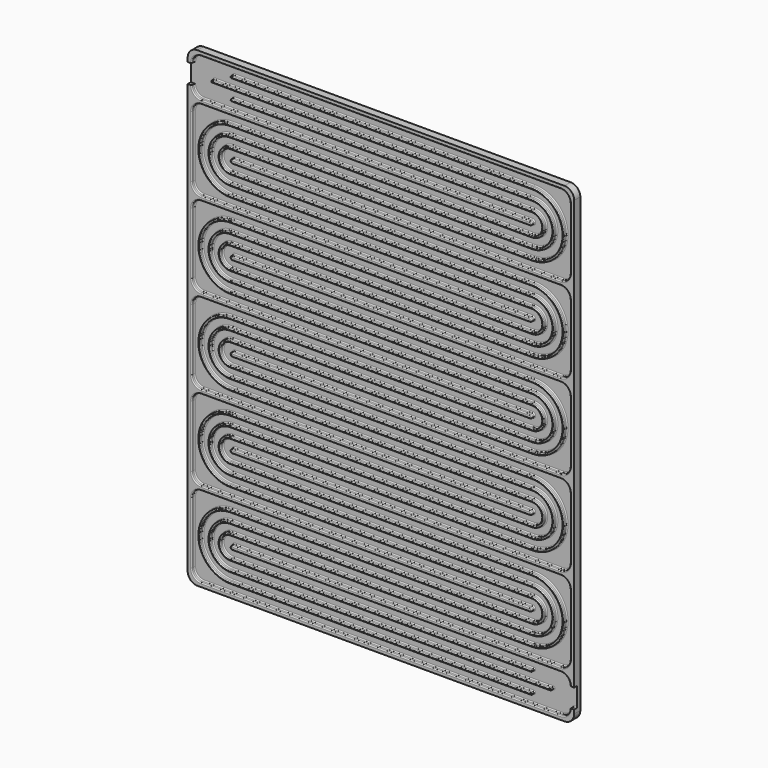
from build123d import *

# Parameters (mm, degrees)
F1_DEPTH = 4
F3_DEPTH = 2
F4_W     = 156
F4_H     = 1
F5_DEPTH = 2
F6_R     = 0.49999


# Not quite as in the source:
# - a fillet or chamfer is up to 0.001 mm smaller than in the source, because OpenCascade refuses the exact size


with BuildPart() as f1:
    # F0 (on Front) → F1 (new body)
    with BuildSketch(Plane.XZ):
        with BuildLine():
            ThreePointArc((0, 5), (1.4644660941, 1.4644660941), (5, 0))
            Line((5, 0), (195, 0))
            ThreePointArc((195, 0), (198.5355339059, 1.4644660941), (200, 5))
            Line((200, 5), (200, 239))
            ThreePointArc((200, 239), (198.5355339059, 242.5355339059), (195, 244))
            Line((195, 244), (5, 244))
            ThreePointArc((5, 244), (1.4644660941, 242.5355339059), (0, 239))
            Line((0, 239), (0, 5))
        make_face()
    extrude(amount=F1_DEPTH)

    # F2 (on face) → F3 (cut)
    with BuildSketch(Plane.XZ.offset(4)):
        with BuildLine():
            Line((193, 242), (7, 242))
            ThreePointArc((7, 242), (3.4644660941, 240.5355339059), (2, 237))
            Line((2, 237), (0, 237))
            Line((0, 237), (0, 227))
            Line((0, 227), (2, 227))
            ThreePointArc((2, 227), (3.4644660941, 223.4644660941), (7, 222))
            Line((7, 222), (177, 222))
            ThreePointArc((177, 222), (177.7071067812, 221.7071067812), (178, 221))
            ThreePointArc((178, 221), (177.7071067812, 220.2928932188), (177, 220))
            Line((177, 220), (7, 220))
            ThreePointArc((7, 220), (3.4644660941, 218.5355339059), (2, 215))
            Line((2, 215), (2, 183))
            ThreePointArc((2, 183), (3.4644660941, 179.4644660941), (7, 178))
            Line((7, 178), (177, 178))
            ThreePointArc((177, 178), (177.7071067812, 177.7071067812), (178, 177))
            ThreePointArc((178, 177), (177.7071067812, 176.2928932188), (177, 176))
            Line((177, 176), (7, 176))
            ThreePointArc((7, 176), (3.4644660941, 174.5355339059), (2, 171))
            Line((2, 171), (2, 139))
            ThreePointArc((2, 139), (3.4644660941, 135.4644660941), (7, 134))
            Line((7, 134), (177, 134))
            ThreePointArc((177, 134), (177.7071067812, 133.7071067812), (178, 133))
            ThreePointArc((178, 133), (177.7071067812, 132.2928932188), (177, 132))
            Line((177, 132), (7, 132))
            ThreePointArc((7, 132), (3.4644660941, 130.5355339059), (2, 127))
            Line((2, 127), (2, 95))
            ThreePointArc((2, 95), (3.4644660941, 91.4644660941), (7, 90))
            Line((7, 90), (177, 90))
            ThreePointArc((177, 90), (177.7071067812, 89.7071067812), (178, 89))
            ThreePointArc((178, 89), (177.7071067812, 88.2928932188), (177, 88))
            Line((177, 88), (7, 88))
            ThreePointArc((7, 88), (3.4644660941, 86.5355339059), (2, 83))
            Line((2, 83), (2, 51))
            ThreePointArc((2, 51), (3.4644660941, 47.4644660941), (7, 46))
            Line((7, 46), (177, 46))
            ThreePointArc((177, 46), (177.7071067812, 45.7071067812), (178, 45))
            ThreePointArc((178, 45), (177.7071067812, 44.2928932188), (177, 44))
            Line((177, 44), (6.8, 44))
            ThreePointArc((6.8, 44), (3.4058874503, 42.5941125497), (2, 39.2))
            Line((2, 39.2), (2, 7))
            ThreePointArc((2, 7), (3.4644660941, 3.4644660941), (7, 2))
            Line((7, 2), (193, 2))
            ThreePointArc((193, 2), (196.5355339059, 3.4644660941), (198, 7))
            Line((198, 7), (200, 7))
            Line((200, 7), (200, 17))
            Line((200, 17), (198, 17))
            ThreePointArc((198, 17), (196.5355339059, 20.5355339059), (193, 22))
            Line((193, 22), (23, 22))
            ThreePointArc((23, 22), (22.2928932188, 22.2928932188), (22, 23))
            ThreePointArc((22, 23), (22.2928932188, 23.7071067812), (23, 24))
            Line((23, 24), (193, 24))
            ThreePointArc((193, 24), (196.5355339059, 25.4644660941), (198, 29))
            Line((198, 29), (198, 61))
            ThreePointArc((198, 61), (196.5355339059, 64.5355339059), (193, 66))
            Line((193, 66), (23, 66))
            ThreePointArc((23, 66), (22.2928932188, 66.2928932188), (22, 67))
            ThreePointArc((22, 67), (22.2928932188, 67.7071067812), (23, 68))
            Line((23, 68), (193, 68))
            ThreePointArc((193, 68), (196.5355339059, 69.4644660941), (198, 73))
            Line((198, 73), (198, 105))
            ThreePointArc((198, 105), (196.5355339059, 108.5355339059), (193, 110))
            Line((193, 110), (23, 110))
            ThreePointArc((23, 110), (22.2928932188, 110.2928932188), (22, 111))
            ThreePointArc((22, 111), (22.2928932188, 111.7071067812), (23, 112))
            Line((23, 112), (193, 112))
            ThreePointArc((193, 112), (196.5355339059, 113.4644660941), (198, 117))
            Line((198, 117), (198, 149))
            ThreePointArc((198, 149), (196.5355339059, 152.5355339059), (193, 154))
            Line((193, 154), (23, 154))
            ThreePointArc((23, 154), (22.2928932188, 154.2928932188), (22, 155))
            ThreePointArc((22, 155), (22.2928932188, 155.7071067812), (23, 156))
            Line((23, 156), (193, 156))
            ThreePointArc((193, 156), (196.5355339059, 157.4644660941), (198, 161))
            Line((198, 161), (198, 193))
            ThreePointArc((198, 193), (196.5355339059, 196.5355339059), (193, 198))
            Line((193, 198), (23, 198))
            ThreePointArc((23, 198), (22.2928932188, 198.2928932188), (22, 199))
            ThreePointArc((22, 199), (22.2928932188, 199.7071067812), (23, 200))
            Line((23, 200), (193, 200))
            ThreePointArc((193, 200), (196.5355339059, 201.4644660941), (198, 205))
            Line((198, 205), (198, 237))
            ThreePointArc((198, 237), (196.5355339059, 240.5355339059), (193, 242))
        make_face()
    extrude(amount=-F3_DEPTH, mode=Mode.SUBTRACT)

    # F4 (on face) → F5 (join)
    with BuildSketch(Plane.XZ.offset(2)):
        with Locations((100, 6.75)):
            Rectangle(F4_W, F4_H)
        with BuildLine():
            Line((22, 6.25), (22, 7.25))
            ThreePointArc((22, 7.25), (6.25, 23), (22, 38.75))
            Line((22, 38.75), (178, 38.75))
            ThreePointArc((178, 38.75), (184.25, 45), (178, 51.25))
            Line((178, 51.25), (22, 51.25))
            Line((22, 51.25), (22, 50.25))
            Line((22, 50.25), (178, 50.25))
            ThreePointArc((178, 50.25), (183.25, 45), (178, 39.75))
            Line((178, 39.75), (22, 39.75))
            ThreePointArc((22, 39.75), (5.25, 23), (22, 6.25))
        make_face()
        with BuildLine():
            Line((22, 50.25), (22, 51.25))
            ThreePointArc((22, 51.25), (6.25, 67), (22, 82.75))
            Line((22, 82.75), (22, 83.75))
            ThreePointArc((22, 83.75), (5.25, 67), (22, 50.25))
        make_face()
        with Locations((100, 83.25)):
            Rectangle(F4_W, F4_H)
        with BuildLine():
            Line((178, 83.75), (178, 82.75))
            ThreePointArc((178, 82.75), (184.25, 89), (178, 95.25))
            Line((178, 95.25), (178, 94.25))
            ThreePointArc((178, 94.25), (183.25, 89), (178, 83.75))
        make_face()
        with Locations((100, 94.75)):
            Rectangle(F4_W, F4_H)
        with BuildLine():
            Line((22, 94.25), (22, 95.25))
            ThreePointArc((22, 95.25), (6.25, 111), (22, 126.75))
            Line((22, 126.75), (22, 127.75))
            ThreePointArc((22, 127.75), (5.25, 111), (22, 94.25))
        make_face()
        with Locations((100, 127.25)):
            Rectangle(F4_W, F4_H)
        with BuildLine():
            Line((178, 127.75), (178, 126.75))
            ThreePointArc((178, 126.75), (184.25, 133), (178, 139.25))
            Line((178, 139.25), (178, 138.25))
            ThreePointArc((178, 138.25), (183.25, 133), (178, 127.75))
        make_face()
        with Locations((100, 138.75)):
            Rectangle(F4_W, F4_H)
        with BuildLine():
            Line((22, 138.25), (22, 139.25))
            ThreePointArc((22, 139.25), (6.25, 155), (22, 170.75))
            Line((22, 170.75), (22, 171.75))
            ThreePointArc((22, 171.75), (5.25, 155), (22, 138.25))
        make_face()
        with Locations((100, 171.25)):
            Rectangle(F4_W, F4_H)
        with BuildLine():
            Line((178, 171.75), (178, 170.75))
            ThreePointArc((178, 170.75), (184.25, 177), (178, 183.25))
            Line((178, 183.25), (178, 182.25))
            ThreePointArc((178, 182.25), (183.25, 177), (178, 171.75))
        make_face()
        with Locations((100, 182.75)):
            Rectangle(F4_W, F4_H)
        with BuildLine():
            Line((22, 182.25), (22, 183.25))
            ThreePointArc((22, 183.25), (6.25, 199), (22, 214.75))
            Line((22, 214.75), (22, 215.75))
            ThreePointArc((22, 215.75), (5.25, 199), (22, 182.25))
        make_face()
        with Locations((100, 215.25)):
            Rectangle(F4_W, F4_H)
        with BuildLine():
            Line((178, 215.75), (178, 214.75))
            ThreePointArc((178, 214.75), (184.25, 221), (178, 227.25))
            Line((178, 227.25), (178, 226.25))
            ThreePointArc((178, 226.25), (183.25, 221), (178, 215.75))
        make_face()
        with Locations((100, 226.75)):
            Rectangle(F4_W, F4_H)
        Polygon((178, 12.5), (22, 12.5), (22, 11.5), (178, 11.5), (188, 11.5), (188, 12.5), align=None)
        with BuildLine():
            Line((22, 11.5), (22, 12.5))
            ThreePointArc((22, 12.5), (11.5, 23), (22, 33.5))
            Line((22, 33.5), (178, 33.5))
            ThreePointArc((178, 33.5), (189.5, 45), (178, 56.5))
            Line((178, 56.5), (22, 56.5))
            Line((22, 56.5), (22, 55.5))
            Line((22, 55.5), (178, 55.5))
            ThreePointArc((178, 55.5), (188.5, 45), (178, 34.5))
            Line((178, 34.5), (22, 34.5))
            ThreePointArc((22, 34.5), (10.5, 23), (22, 11.5))
        make_face()
        with BuildLine():
            Line((22, 55.5), (22, 56.5))
            ThreePointArc((22, 56.5), (11.5, 67), (22, 77.5))
            Line((22, 77.5), (22, 78.5))
            ThreePointArc((22, 78.5), (10.5, 67), (22, 55.5))
        make_face()
        with Locations((100, 78)):
            Rectangle(F4_W, F4_H)
        with BuildLine():
            Line((178, 78.5), (178, 77.5))
            ThreePointArc((178, 77.5), (189.5, 89), (178, 100.5))
            Line((178, 100.5), (178, 99.5))
            ThreePointArc((178, 99.5), (188.5, 89), (178, 78.5))
        make_face()
        with Locations((100, 100)):
            Rectangle(F4_W, F4_H)
        with BuildLine():
            Line((22, 99.5), (22, 100.5))
            ThreePointArc((22, 100.5), (11.5, 111), (22, 121.5))
            Line((22, 121.5), (22, 122.5))
            ThreePointArc((22, 122.5), (10.5, 111), (22, 99.5))
        make_face()
        with Locations((100, 122)):
            Rectangle(F4_W, F4_H)
        with BuildLine():
            Line((178, 122.5), (178, 121.5))
            ThreePointArc((178, 121.5), (189.5, 133), (178, 144.5))
            Line((178, 144.5), (178, 143.5))
            ThreePointArc((178, 143.5), (188.5, 133), (178, 122.5))
        make_face()
        with Locations((100, 144)):
            Rectangle(F4_W, F4_H)
        with BuildLine():
            Line((22, 143.5), (22, 144.5))
            ThreePointArc((22, 144.5), (11.5, 155), (22, 165.5))
            Line((22, 165.5), (22, 166.5))
            ThreePointArc((22, 166.5), (10.5, 155), (22, 143.5))
        make_face()
        with Locations((100, 166)):
            Rectangle(F4_W, F4_H)
        with BuildLine():
            Line((178, 166.5), (178, 165.5))
            ThreePointArc((178, 165.5), (189.5, 177), (178, 188.5))
            Line((178, 188.5), (178, 187.5))
            ThreePointArc((178, 187.5), (188.5, 177), (178, 166.5))
        make_face()
        with Locations((100, 188)):
            Rectangle(F4_W, F4_H)
        with BuildLine():
            Line((22, 187.5), (22, 188.5))
            ThreePointArc((22, 188.5), (11.5, 199), (22, 209.5))
            Line((22, 209.5), (22, 210.5))
            ThreePointArc((22, 210.5), (10.5, 199), (22, 187.5))
        make_face()
        with Locations((100, 210)):
            Rectangle(F4_W, F4_H)
        with BuildLine():
            Line((178, 210.5), (178, 209.5))
            ThreePointArc((178, 209.5), (189.5, 221), (178, 232.5))
            Line((178, 232.5), (178, 231.5))
            ThreePointArc((178, 231.5), (188.5, 221), (178, 210.5))
        make_face()
        Polygon((178, 231.5), (178, 232.5), (22, 232.5), (12, 232.5), (12, 231.5), (22, 231.5), align=None)
        with Locations((100, 17.25)):
            Rectangle(F4_W, F4_H)
        with BuildLine():
            Line((22, 16.75), (22, 17.75))
            ThreePointArc((22, 17.75), (16.75, 23), (22, 28.25))
            Line((22, 28.25), (22, 29.25))
            ThreePointArc((22, 29.25), (15.75, 23), (22, 16.75))
        make_face()
        with BuildLine():
            Line((22, 29.25), (22, 28.25))
            Line((22, 28.25), (178, 28.25))
            ThreePointArc((178, 28.25), (194.75, 45), (178, 61.75))
            Line((178, 61.75), (22, 61.75))
            Line((22, 61.75), (22, 60.75))
            Line((22, 60.75), (178, 60.75))
            ThreePointArc((178, 60.75), (193.75, 45), (178, 29.25))
            Line((178, 29.25), (22, 29.25))
        make_face()
        with BuildLine():
            Line((22, 60.75), (22, 61.75))
            ThreePointArc((22, 61.75), (16.75, 67), (22, 72.25))
            Line((22, 72.25), (22, 73.25))
            ThreePointArc((22, 73.25), (15.75, 67), (22, 60.75))
        make_face()
        with Locations((100, 72.75)):
            Rectangle(F4_W, F4_H)
        with BuildLine():
            Line((178, 73.25), (178, 72.25))
            ThreePointArc((178, 72.25), (194.75, 89), (178, 105.75))
            Line((178, 105.75), (178, 104.75))
            ThreePointArc((178, 104.75), (193.75, 89), (178, 73.25))
        make_face()
        with Locations((100, 105.25)):
            Rectangle(F4_W, F4_H)
        with BuildLine():
            Line((22, 104.75), (22, 105.75))
            ThreePointArc((22, 105.75), (16.75, 111), (22, 116.25))
            Line((22, 116.25), (22, 117.25))
            ThreePointArc((22, 117.25), (15.75, 111), (22, 104.75))
        make_face()
        with Locations((100, 116.75)):
            Rectangle(F4_W, F4_H)
        with BuildLine():
            Line((178, 117.25), (178, 116.25))
            ThreePointArc((178, 116.25), (194.75, 133), (178, 149.75))
            Line((178, 149.75), (178, 148.75))
            ThreePointArc((178, 148.75), (193.75, 133), (178, 117.25))
        make_face()
        with Locations((100, 149.25)):
            Rectangle(F4_W, F4_H)
        with BuildLine():
            Line((22, 148.75), (22, 149.75))
            ThreePointArc((22, 149.75), (16.75, 155), (22, 160.25))
            Line((22, 160.25), (22, 161.25))
            ThreePointArc((22, 161.25), (15.75, 155), (22, 148.75))
        make_face()
        with Locations((100, 160.75)):
            Rectangle(F4_W, F4_H)
        with BuildLine():
            Line((178, 161.25), (178, 160.25))
            ThreePointArc((178, 160.25), (194.75, 177), (178, 193.75))
            Line((178, 193.75), (178, 192.75))
            ThreePointArc((178, 192.75), (193.75, 177), (178, 161.25))
        make_face()
        with Locations((100, 193.25)):
            Rectangle(F4_W, F4_H)
        with BuildLine():
            Line((22, 192.75), (22, 193.75))
            ThreePointArc((22, 193.75), (16.75, 199), (22, 204.25))
            Line((22, 204.25), (22, 205.25))
            ThreePointArc((22, 205.25), (15.75, 199), (22, 192.75))
        make_face()
        with Locations((100, 204.75)):
            Rectangle(F4_W, F4_H)
        with BuildLine():
            Line((178, 205.25), (178, 204.25))
            ThreePointArc((178, 204.25), (194.75, 221), (178, 237.75))
            Line((178, 237.75), (178, 236.75))
            ThreePointArc((178, 236.75), (193.75, 221), (178, 205.25))
        make_face()
        with Locations((100, 237.25)):
            Rectangle(F4_W, F4_H)
    extrude(amount=F5_DEPTH)

    # F6 (radius 0.5 in the source; OpenCascade refuses exactly that, so slightly less here)
    f6_edges = [f1.edges().sort_by_distance(p)[0] for p in [
        (7, -3, 90),
        (177, -3, 90),
        (92, -4, 90),
        (92, -2, 90),
        (23, -3, 68),
        (193, -3, 68),
        (108, -4, 68),
        (108, -2, 68),
        (193, -3, 66),
        (23, -3, 66),
        (108, -4, 66),
        (108, -2, 66),
        (193, -3, 242),
        (7, -3, 242),
        (100, -4, 242),
        (100, -2, 242),
        (198, -3, 205),
        (198, -3, 237),
        (198, -4, 221),
        (198, -2, 221),
        (196.535534, -4, 240.535534),
        (196.535534, -2, 240.535534),
        (7, -3, 46),
        (177, -3, 46),
        (92, -4, 46),
        (92, -2, 46),
        (177, -3, 44),
        (6.8, -3, 44),
        (91.9, -4, 44),
        (91.9, -2, 44),
        (23, -3, 24),
        (193, -3, 24),
        (108, -4, 24),
        (108, -2, 24),
        (193, -3, 22),
        (23, -3, 22),
        (108, -4, 22),
        (108, -2, 22),
        (177, -3, 88),
        (7, -3, 88),
        (92, -4, 88),
        (92, -2, 88),
        (178, -3, 29.25),
        (22, -3, 29.25),
        (100, -2, 29.25),
        (100, -4, 29.25),
        (178, -3, 16.75),
        (178, -3, 17.75),
        (178, -2, 17.25),
        (178, -4, 17.25),
        (22, -3, 38.75),
        (178, -3, 38.75),
        (100, -2, 38.75),
        (100, -4, 38.75),
        (178, -3, 7.25),
        (22, -3, 7.25),
        (100, -2, 7.25),
        (100, -4, 7.25),
        (6.25, -4, 23),
        (184.25, -4, 45),
        (100, -4, 51.25),
        (6.25, -4, 67),
        (100, -4, 82.75),
        (184.25, -4, 89),
        (100, -4, 95.25),
        (6.25, -4, 111),
        (100, -4, 126.75),
        (184.25, -4, 133),
        (100, -4, 139.25),
        (6.25, -4, 155),
        (100, -4, 170.75),
        (184.25, -4, 177),
        (100, -4, 183.25),
        (6.25, -4, 199),
        (100, -4, 214.75),
        (184.25, -4, 221),
        (100, -4, 227.25),
        (22, -4, 226.75),
        (100, -4, 226.25),
        (183.25, -4, 221),
        (100, -4, 215.75),
        (5.25, -4, 199),
        (100, -4, 182.25),
        (183.25, -4, 177),
        (100, -4, 171.75),
        (5.25, -4, 155),
        (100, -4, 138.25),
        (183.25, -4, 133),
        (100, -4, 127.75),
        (5.25, -4, 111),
        (100, -4, 94.25),
        (183.25, -4, 89),
        (100, -4, 83.75),
        (5.25, -4, 67),
        (100, -4, 50.25),
        (183.25, -4, 45),
        (100, -4, 39.75),
        (5.25, -4, 23),
        (100, -4, 6.25),
        (178, -4, 6.75),
        (11.5, -4, 23),
        (100, -4, 33.5),
        (189.5, -4, 45),
        (100, -4, 56.5),
        (11.5, -4, 67),
        (100, -4, 77.5),
        (189.5, -4, 89),
        (100, -4, 100.5),
        (11.5, -4, 111),
        (100, -4, 121.5),
        (189.5, -4, 133),
        (100, -4, 144.5),
        (11.5, -4, 155),
        (100, -4, 165.5),
        (189.5, -4, 177),
        (100, -4, 188.5),
        (11.5, -4, 199),
        (100, -4, 209.5),
        (189.5, -4, 221),
        (95, -4, 232.5),
        (12, -4, 232),
        (95, -4, 231.5),
        (188.5, -4, 221),
        (100, -4, 210.5),
        (10.5, -4, 199),
        (100, -4, 187.5),
        (188.5, -4, 177),
        (100, -4, 166.5),
        (10.5, -4, 155),
        (100, -4, 143.5),
        (188.5, -4, 133),
        (100, -4, 122.5),
        (10.5, -4, 111),
        (100, -4, 99.5),
        (188.5, -4, 89),
        (100, -4, 78.5),
        (10.5, -4, 67),
        (100, -4, 55.5),
        (188.5, -4, 45),
        (100, -4, 34.5),
        (10.5, -4, 23),
        (105, -4, 11.5),
        (188, -4, 12),
        (105, -4, 12.5),
        (188, -3, 12.5),
        (22, -3, 12.5),
        (105, -2, 12.5),
        (22, -3, 11.5),
        (188, -3, 11.5),
        (105, -2, 11.5),
        (22, -3, 17.75),
        (100, -2, 17.75),
        (100, -4, 17.75),
        (16.75, -4, 23),
        (100, -4, 28.25),
        (194.75, -4, 45),
        (100, -4, 61.75),
        (16.75, -4, 67),
        (100, -4, 72.25),
        (194.75, -4, 89),
        (100, -4, 105.75),
        (16.75, -4, 111),
        (100, -4, 116.25),
        (194.75, -4, 133),
        (100, -4, 149.75),
        (16.75, -4, 155),
        (100, -4, 160.25),
        (194.75, -4, 177),
        (100, -4, 193.75),
        (16.75, -4, 199),
        (100, -4, 204.25),
        (194.75, -4, 221),
        (100, -4, 237.75),
        (22, -4, 237.25),
        (100, -4, 236.75),
        (193.75, -4, 221),
        (100, -4, 205.25),
        (15.75, -4, 199),
        (100, -4, 192.75),
        (193.75, -4, 177),
        (100, -4, 161.25),
        (15.75, -4, 155),
        (100, -4, 148.75),
        (193.75, -4, 133),
        (100, -4, 117.25),
        (15.75, -4, 111),
        (100, -4, 104.75),
        (193.75, -4, 89),
        (100, -4, 73.25),
        (15.75, -4, 67),
        (100, -4, 60.75),
        (193.75, -4, 45),
        (15.75, -4, 23),
        (100, -4, 16.75),
        (22, -3, 16.75),
        (100, -2, 16.75),
        (23, -3, 200),
        (193, -3, 200),
        (108, -4, 200),
        (108, -2, 200),
        (198, -3, 105),
        (193, -3, 110),
        (196.535534, -4, 108.535534),
        (196.535534, -2, 108.535534),
        (193, -3, 112),
        (198, -3, 117),
        (196.535534, -4, 113.464466),
        (196.535534, -2, 113.464466),
        (177, -3, 220),
        (7, -3, 220),
        (92, -4, 220),
        (92, -2, 220),
        (198, -3, 73),
        (198, -4, 89),
        (198, -2, 89),
        (198, -3, 149),
        (193, -3, 154),
        (196.535534, -4, 152.535534),
        (196.535534, -2, 152.535534),
        (193, -3, 198),
        (23, -3, 198),
        (108, -4, 198),
        (108, -2, 198),
        (196.535534, -4, 69.464466),
        (196.535534, -2, 69.464466),
        (7, -3, 222),
        (177, -3, 222),
        (92, -4, 222),
        (92, -2, 222),
        (198, -3, 29),
        (196.535534, -4, 25.464466),
        (196.535534, -2, 25.464466),
        (196.535534, -4, 64.535534),
        (177, -3, 132),
        (7, -3, 132),
        (92, -4, 132),
        (92, -2, 132),
        (23, -3, 112),
        (108, -4, 112),
        (108, -2, 112),
        (196.535534, -4, 20.535534),
        (23, -3, 110),
        (108, -4, 110),
        (108, -2, 110),
        (7, -3, 134),
        (177, -3, 134),
        (92, -4, 134),
        (92, -2, 134),
        (198, -3, 61),
        (196.535534, -2, 64.535534),
        (198, -3, 17),
        (196.535534, -2, 20.535534),
        (177, -3, 176),
        (7, -3, 176),
        (92, -4, 176),
        (92, -2, 176),
        (23, -3, 156),
        (193, -3, 156),
        (108, -4, 156),
        (108, -2, 156),
        (198, -4, 45),
        (198, -2, 45),
        (23, -3, 154),
        (108, -4, 154),
        (108, -2, 154),
        (198, -3, 161),
        (198, -3, 193),
        (198, -4, 177),
        (198, -2, 177),
        (196.535534, -4, 201.464466),
        (196.535534, -2, 201.464466),
        (7, -3, 178),
        (177, -3, 178),
        (92, -4, 178),
        (92, -2, 178),
        (198, -4, 133),
        (198, -2, 133),
        (196.535534, -4, 196.535534),
        (196.535534, -2, 196.535534),
        (196.535534, -4, 157.464466),
        (196.535534, -2, 157.464466),
        (22, -3, 77.5),
        (178, -3, 77.5),
        (100, -2, 77.5),
        (22, -3, 138.25),
        (178, -3, 138.25),
        (100, -2, 138.25),
        (178, -3, 205.25),
        (22, -3, 205.25),
        (100, -2, 205.25),
        (22, -3, 34.5),
        (10.5, -2, 23),
        (22, -3, 161.25),
        (22, -3, 148.75),
        (15.75, -2, 155),
        (178, -3, 28.25),
        (178, -3, 61.75),
        (194.75, -2, 45),
        (22, -3, 72.25),
        (178, -3, 72.25),
        (100, -2, 72.25),
        (178, -3, 139.25),
        (22, -3, 139.25),
        (100, -2, 139.25),
        (22, -3, 187.5),
        (178, -3, 187.5),
        (100, -2, 187.5),
        (15.75, -2, 23),
        (178, -3, 33.5),
        (178, -3, 56.5),
        (189.5, -2, 45),
        (178, -3, 126.75),
        (184.25, -2, 133),
        (178, -3, 144.5),
        (22, -3, 144.5),
        (100, -2, 144.5),
        (22, -3, 214.75),
        (178, -3, 214.75),
        (100, -2, 214.75),
        (22, -3, 171.75),
        (5.25, -2, 155),
        (178, -3, 34.5),
        (100, -2, 34.5),
        (178, -3, 149.75),
        (22, -3, 149.75),
        (100, -2, 149.75),
        (22, -3, 166.5),
        (22, -3, 143.5),
        (10.5, -2, 155),
        (188, -2, 12),
        (178, -3, 160.25),
        (178, -3, 193.75),
        (194.75, -2, 177),
        (178, -3, 95.25),
        (22, -3, 95.25),
        (100, -2, 95.25),
        (178, -3, 143.5),
        (100, -2, 143.5),
        (22, -3, 204.25),
        (178, -3, 204.25),
        (100, -2, 204.25),
        (22, -3, 39.75),
        (22, -3, 6.25),
        (5.25, -2, 23),
        (178, -3, 100.5),
        (22, -3, 100.5),
        (100, -2, 100.5),
        (22, -3, 170.75),
        (178, -3, 170.75),
        (100, -2, 170.75),
        (178, -3, 215.75),
        (22, -3, 215.75),
        (100, -2, 215.75),
        (22, -3, 83.75),
        (22, -3, 50.25),
        (5.25, -2, 67),
        (178, -3, 165.5),
        (178, -3, 188.5),
        (189.5, -2, 177),
        (22, -3, 33.5),
        (100, -2, 33.5),
        (22, -3, 94.25),
        (178, -3, 94.25),
        (100, -2, 94.25),
        (178, -3, 161.25),
        (100, -2, 161.25),
        (22, -3, 209.5),
        (178, -3, 209.5),
        (100, -2, 209.5),
        (22, -3, 73.25),
        (22, -3, 60.75),
        (15.75, -2, 67),
        (178, -3, 183.25),
        (184.25, -2, 177),
        (22, -3, 236.75),
        (178, -3, 236.75),
        (100, -2, 236.75),
        (22, -3, 78.5),
        (22, -3, 55.5),
        (10.5, -2, 67),
        (22, -3, 182.25),
        (5.25, -2, 199),
        (178, -3, 105.75),
        (194.75, -2, 89),
        (178, -3, 51.25),
        (22, -3, 51.25),
        (100, -2, 51.25),
        (22, -3, 99.5),
        (178, -3, 99.5),
        (100, -2, 99.5),
        (22, -3, 160.25),
        (100, -2, 160.25),
        (178, -3, 227.25),
        (22, -3, 227.25),
        (100, -2, 227.25),
        (22, -3, 192.75),
        (15.75, -2, 199),
        (22, -3, 56.5),
        (100, -2, 56.5),
        (22, -3, 126.75),
        (100, -2, 126.75),
        (178, -3, 171.75),
        (100, -2, 171.75),
        (22, -3, 210.5),
        (10.5, -2, 199),
        (189.5, -2, 89),
        (178, -3, 237.75),
        (194.75, -2, 221),
        (178, -3, 50.25),
        (100, -2, 50.25),
        (178, -3, 117.25),
        (22, -3, 117.25),
        (100, -2, 117.25),
        (22, -3, 165.5),
        (100, -2, 165.5),
        (22, -3, 226.25),
        (178, -3, 226.25),
        (100, -2, 226.25),
        (178, -3, 82.75),
        (184.25, -2, 89),
        (178, -3, 122.5),
        (22, -3, 122.5),
        (100, -2, 122.5),
        (178, -3, 192.75),
        (100, -2, 192.75),
        (22, -3, 237.75),
        (100, -2, 237.75),
        (22, -3, 127.75),
        (5.25, -2, 111),
        (178, -3, 232.5),
        (189.5, -2, 221),
        (178, -3, 55.5),
        (100, -2, 55.5),
        (22, -3, 116.25),
        (178, -3, 116.25),
        (100, -2, 116.25),
        (22, -3, 183.25),
        (100, -2, 183.25),
        (22, -3, 104.75),
        (15.75, -2, 111),
        (184.25, -2, 221),
        (178, -3, 127.75),
        (100, -2, 127.75),
        (22, -2, 237.25),
        (10.5, -2, 111),
        (194.75, -2, 133),
        (178, -3, 73.25),
        (100, -2, 73.25),
        (22, -3, 121.5),
        (178, -3, 121.5),
        (100, -2, 121.5),
        (178, -3, 182.25),
        (100, -2, 182.25),
        (22, -2, 226.75),
        (184.25, -2, 45),
        (178, -3, 78.5),
        (100, -2, 78.5),
        (178, -3, 148.75),
        (100, -2, 148.75),
        (22, -3, 193.75),
        (100, -2, 193.75),
        (189.5, -2, 133),
        (178, -3, 6.25),
        (100, -2, 6.25),
        (22, -4, 155),
        (178, -4, 177),
        (22, -4, 111),
        (178, -4, 133),
        (22, -4, 67),
        (178, -4, 89),
        (178, -4, 45),
        (22, -4, 199),
        (178, -4, 221),
        (193.75, -2, 177),
        (6.25, -2, 111),
        (178, -3, 83.75),
        (100, -2, 83.75),
        (11.5, -2, 23),
        (178, -3, 60.75),
        (193.75, -2, 45),
        (183.25, -2, 177),
        (178, -3, 104.75),
        (100, -2, 104.75),
        (178, -3, 210.5),
        (100, -2, 210.5),
        (6.25, -2, 23),
        (22, -3, 28.25),
        (100, -2, 28.25),
        (11.5, -2, 155),
        (12, -3, 232.5),
        (12, -3, 231.5),
        (12, -2, 232),
        (178, -3, 166.5),
        (188.5, -2, 177),
        (178, -3, 39.75),
        (100, -2, 39.75),
        (16.75, -2, 155),
        (183.25, -2, 89),
        (6.25, -2, 155),
        (193.75, -2, 89),
        (100, -2, 60.75),
        (22, -3, 105.75),
        (100, -2, 105.75),
        (100, -2, 166.5),
        (183.25, -2, 221),
        (11.5, -2, 67),
        (188.5, -2, 89),
        (193.75, -2, 221),
        (95, -2, 232.5),
        (22, -3, 61.75),
        (16.75, -2, 67),
        (22, -3, 82.75),
        (6.25, -2, 67),
        (22, -3, 188.5),
        (11.5, -2, 199),
        (178, -3, 231.5),
        (188.5, -2, 221),
        (100, -2, 61.75),
        (16.75, -2, 199),
        (183.25, -2, 133),
        (6.25, -2, 199),
        (193.75, -2, 133),
        (100, -2, 188.5),
        (11.5, -2, 111),
        (188.5, -2, 133),
        (16.75, -2, 23),
        (16.75, -2, 111),
        (188.5, -2, 45),
        (178, -2, 45),
        (178, -2, 6.75),
        (198, -3, 7),
        (22, -2, 67),
        (22, -2, 199),
        (22, -2, 111),
        (22, -4, 23),
        (22, -2, 155),
        (95, -2, 231.5),
        (100, -2, 82.75),
        (183.25, -2, 45),
        (22, -2, 23),
        (178, -2, 177),
        (178, -2, 89),
        (178, -2, 221),
        (178, -2, 133),
        (3.464466, -4, 223.464466),
        (3.464466, -4, 218.535534),
        (2, -4, 199),
        (3.464466, -4, 179.464466),
        (3.464466, -4, 174.535534),
        (2, -4, 155),
        (3.464466, -4, 135.464466),
        (3.464466, -4, 130.535534),
        (2, -4, 111),
        (3.464466, -4, 91.464466),
        (3.464466, -4, 86.535534),
        (2, -4, 67),
        (3.464466, -4, 47.464466),
        (3.405887, -4, 42.594113),
        (2, -4, 23.1),
        (3.464466, -4, 3.464466),
        (100, -4, 2),
        (196.535534, -4, 3.464466),
        (199, -2, 7),
        (196.535534, -2, 3.464466),
        (100, -2, 2),
        (199, -2, 17),
        (3.464466, -2, 3.464466),
        (2, -2, 23.1),
        (3.405887, -2, 42.594113),
        (3.464466, -2, 47.464466),
        (2, -2, 67),
        (3.464466, -2, 86.535534),
        (3.464466, -2, 91.464466),
        (2, -2, 111),
        (3.464466, -2, 130.535534),
        (3.464466, -2, 135.464466),
        (2, -2, 155),
        (3.464466, -2, 174.535534),
        (3.464466, -2, 179.464466),
        (2, -2, 199),
        (3.464466, -2, 218.535534),
        (3.464466, -2, 223.464466),
        (3.464466, -2, 240.535534),
        (3.464466, -4, 240.535534),
    ]]
    fillet(f6_edges, radius=F6_R)


solid = f1.part
